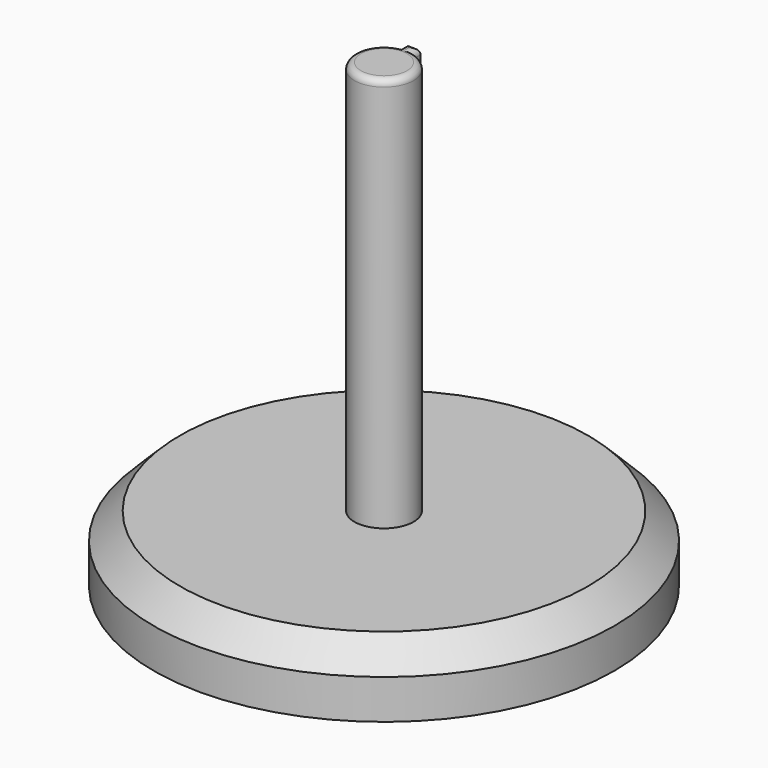
from build123d import *

# Parameters (mm, degrees)
F0_R     = 44.45
F1_DEPTH = 12.7
F2_DEPTH = 88.9
F3_R     = 1.2699
F4_SIZE  = 5.08


# Not quite as in the source:
# - a fillet or chamfer is up to 0.001 mm smaller than in the source, because OpenCascade refuses the exact size


with BuildPart() as f1:
    # F0 (on Top) → F1 (new body)
    with BuildSketch(Plane.XY):
        Circle(F0_R)
        with BuildLine():
            ThreePointArc((1.27, 5.572102386), (0, -5.715), (-1.27, 5.572102386))
            Line((-1.27, 5.572102386), (-1.27, 7.239))
            Line((-1.27, 7.239), (1.27, 7.239))
            Line((1.27, 7.239), (1.27, 5.572102386))
        make_face(mode=Mode.SUBTRACT)
    extrude(amount=F1_DEPTH)

    # F0 (on Top) → F2 (join)
    with BuildSketch(Plane.XY):
        with BuildLine():
            Line((-1.27, 7.239), (-1.27, 5.572102386))
            ThreePointArc((-1.27, 5.572102386), (0, -5.715), (1.27, 5.572102386))
            Line((1.27, 5.572102386), (1.27, 7.239))
            Line((1.27, 7.239), (-1.27, 7.239))
        make_face()
    extrude(amount=F2_DEPTH)

    # F3 (radius 1.27 in the source; OpenCascade refuses exactly that, so slightly less here)
    f3_edges = [f1.edges().sort_by_distance(p)[0] for p in [
        (1.27, 6.405551, 88.9),
        (0, 7.239, 88.9),
        (-1.27, 6.405551, 88.9),
        (0, -5.715, 88.9),
    ]]
    fillet(f3_edges, radius=F3_R)

    # F4
    f4_edges = [f1.edges().sort_by_distance(p)[0] for p in [
        (-44.45, 0, 12.7),
    ]]
    chamfer(f4_edges, length=F4_SIZE)


solid = f1.part
